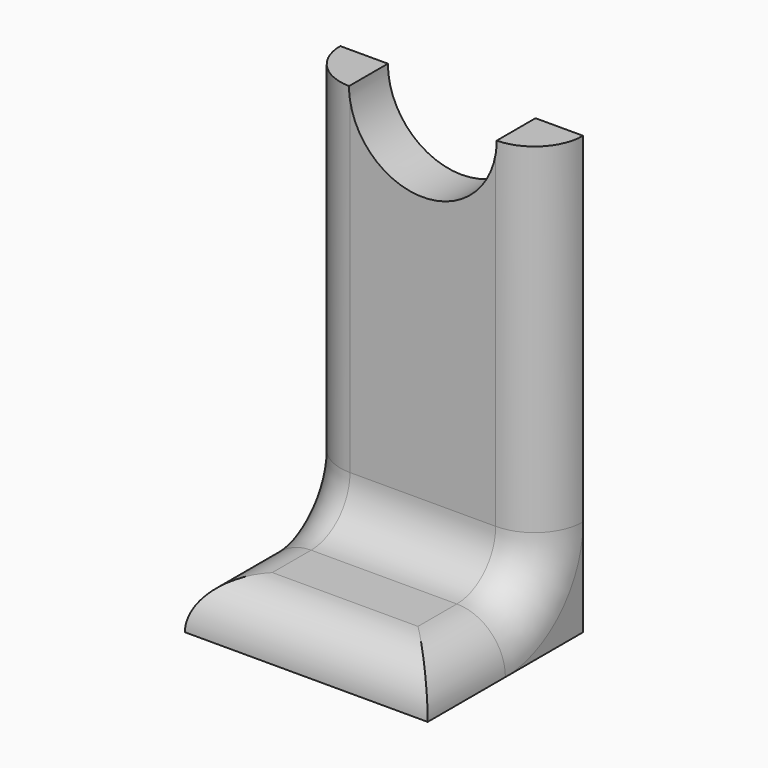
from build123d import *

# Parameters (mm, degrees)
F1_DEPTH = 5
F2_W     = 25
F2_H     = 5
F3_DEPTH = 15
F4_F1_R  = 5
F4_F2_R  = 4.9999


# Not quite as in the source:
# - a fillet or chamfer is up to 0.001 mm smaller than in the source, because OpenCascade refuses the exact size


with BuildPart() as f1:
    # F0 (on Front) → F1 (new body)
    with BuildSketch(Plane.XZ):
        with BuildLine():
            Line((-12.5, -22.5), (12.5, -22.5))
            Line((12.5, -22.5), (12.5, 22.5))
            Line((12.5, 22.5), (7.6, 22.5))
            ThreePointArc((7.6, 22.5), (0, 14.9), (-7.6, 22.5))
            Line((-7.6, 22.5), (-12.5, 22.5))
            Line((-12.5, 22.5), (-12.5, -22.5))
        make_face()
    extrude(amount=F1_DEPTH)

    # F2 (on face) → F3 (join)
    with BuildSketch(Plane.XZ.offset(5)):
        with Locations((0, -20)):
            Rectangle(F2_W, F2_H)
    extrude(amount=F3_DEPTH)

    # F4: fillet of radius 5 on 4 edges, made by hand

    # F4_f1
    f4_f1_edges = [f1.edges().sort_by_distance(p)[0] for p in [
        (0, -5, -17.5),
    ]]
    fillet(f4_f1_edges, radius=F4_F1_R)

    # F4_f2 (radius 5 in the source; OpenCascade refuses exactly that, so slightly less here)
    f4_f2_edges = [f1.edges().sort_by_distance(p)[0] for p in [
        (12.5, -15, -17.5),
        (-12.5, -15, -17.5),
        (0, -20, -17.5),
        (-12.5, -6.4644660941, -16.0355339059),
        (12.5, -6.4644660941, -16.0355339059),
    ]]
    fillet(f4_f2_edges, radius=F4_F2_R)


solid = f1.part
